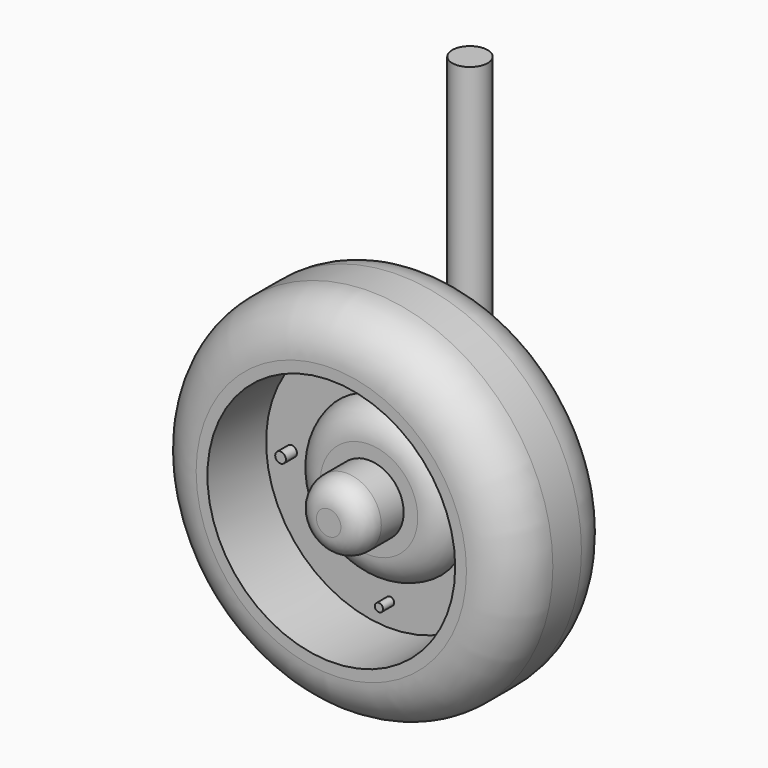
from build123d import *

# Parameters (mm, degrees)
F0_R      = 173.3489517692
F0_R_2    = 117.2606948697
F1_DEPTH  = 124.6887519956
F2_R      = 45.426792545
F3_R      = 121.2481204934
F4_DEPTH  = 55.2671570331
F5_R      = 75.1710071643
F6_DEPTH  = 80.0674576312
F7_R      = 32.7838298789
F8_DEPTH  = 127.7635861188
F9_R      = 21.2247552793
F11_R     = 54.14327209
F12_DEPTH = 72.1452143043
F13_R     = 16.7884886241
F14_DEPTH = 320.553438738
F15_R     = 5.7742203186
F15_R_2   = 5.0578841716
F15_R_3   = 3.8948170444
F15_R_4   = 4.1650665602
F16_DEPTH = 68.3403462172


# Not quite as in the source:
# - a fillet or chamfer that OpenCascade refuses, or shapes differently, is made with other operations: its cross-section is extruded or revolved along the edge and cut away or added


with BuildPart() as f1:
    # F0 (on Front) → F1 (new body)
    with BuildSketch(Plane.XZ):
        Circle(F0_R)
        Circle(F0_R_2, mode=Mode.SUBTRACT)
    extrude(amount=F1_DEPTH)

    # F2
    f2_edges = [f1.edges().sort_by_distance(p)[0] for p in [
        (-173.348952, 0, 0),
        (-173.348952, -124.688752, 0),
    ]]
    fillet(f2_edges, radius=F2_R)

    # F3 (on Front) → F4 (join)
    with BuildSketch(Plane.XZ):
        Circle(F3_R)
    extrude(amount=F4_DEPTH)

    # F5 (on Front) → F6 (join)
    with BuildSketch(Plane.XZ):
        Circle(F5_R)
    extrude(amount=F6_DEPTH)

    # F7 (on Front) → F8 (join)
    with BuildSketch(Plane.XZ):
        Circle(F7_R)
    extrude(amount=F8_DEPTH)

    # F9
    f9_edges = [f1.edges().sort_by_distance(p)[0] for p in [
        (-32.78383, -127.763586, 0),
    ]]
    fillet(f9_edges, radius=F9_R)

    # F10: fillet of radius 29.4120223151 on 1 edges, made by hand

    # F10_s1 → F10_t2 (revolve, cut)
    with BuildSketch(Plane.XY):
        with BuildLine():
            ThreePointArc((46.1227872623, -80.0674576312), (65.2202608468, -73.0240195216), (75.1710071643, -55.2671570331))
            Line((75.1710071643, -55.2671570331), (75.1710071643, -80.0674576312))
            Line((75.1710071643, -80.0674576312), (46.1227872623, -80.0674576312))
        make_face()
    revolve(axis=Axis((0, -80.0674576312, 0), (0, -1, 0)), mode=Mode.SUBTRACT)

    # F11 (on Front) → F12 (join)
    with BuildSketch(Plane.XZ):
        Circle(F11_R)
    extrude(amount=-F12_DEPTH)

    # F13 (on Top) → F14 (join)
    with BuildSketch(Plane.XY):
        with Locations((0, 39.3408536911)):
            Circle(F13_R)
    extrude(amount=F14_DEPTH)

    # F15 (on Front) → F16 (join)
    with BuildSketch(Plane.XZ):
        with Locations((0, 98.4903275967)):
            Circle(F15_R)
        with Locations((-93.0983424187, 0)):
            Circle(F15_R_2)
        with Locations((0, -94.7722494602)):
            Circle(F15_R_3)
        with Locations((95.7255959511, 0)):
            Circle(F15_R_4)
    extrude(amount=F16_DEPTH)


solid = f1.part
